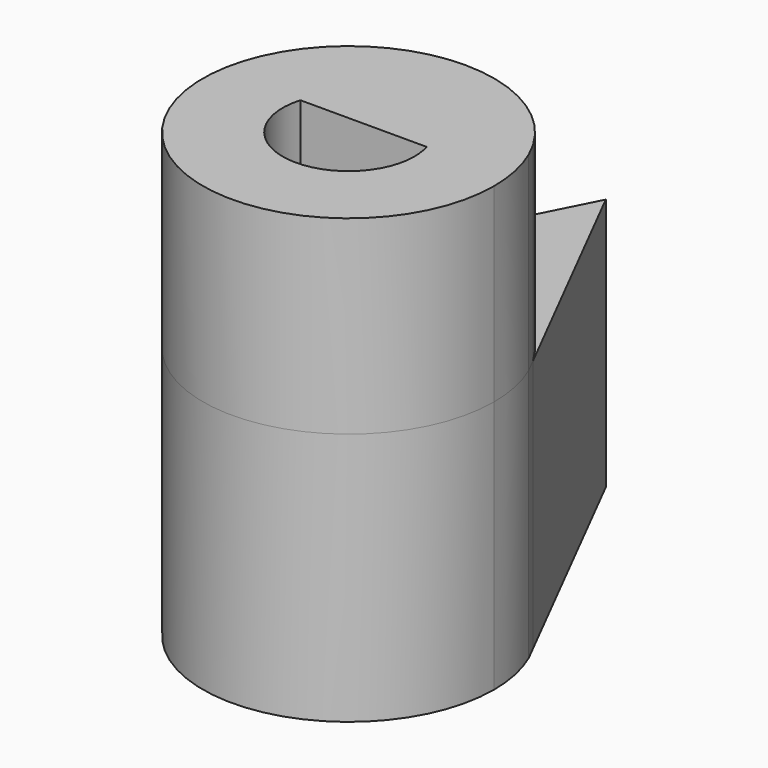
from build123d import *

# Parameters (mm, degrees)
F1_DEPTH = 9.525
F2_DEPTH = 12.7
F3_DEPTH = 9.525


# Not quite as in the source:
# - a feature names something its author has since deleted; it is built from what else it names
# - the program builds the solid bodies; features that only make, move or delete a surface that nothing else refers to are left out


with BuildPart() as f1:
    # F0 (on Top) → F1 (new body)
    with BuildSketch(Plane.XY):
        with BuildLine():
            ThreePointArc((-6.7061053414, 2.890442423), (-1.4756645952, -7.1518473315), (7.3025, 0))
            ThreePointArc((7.3025, 0), (7.1473488528, 1.4973011139), (6.6884881888, 2.9309779936))
            Line((6.6884881888, 2.9309779936), (6.3166219962, 3.6642588347))
            ThreePointArc((6.3166219962, 3.6642588347), (0.0208084361, 7.3024703532), (-6.2956369305, 3.7001975474))
            Line((-6.2956369305, 3.7001975474), (-6.7061053414, 2.890442423))
        make_face()
        with BuildLine():
            ThreePointArc((3.1654351928, 0.9398), (3.2676804469, 0.474835231), (3.302, 0))
            ThreePointArc((3.302, 0), (-0.474835231, -3.2676804469), (-3.1654351928, 0.9398))
            ThreePointArc((-3.1654351928, 0.9398), (0, 3.302), (3.1654351928, 0.9398))
        make_face(mode=Mode.SUBTRACT)
    extrude(amount=F1_DEPTH)

    # F0 (on Top) → F3 (join, through all)
    with BuildSketch(Plane.XY):
        with BuildLine():
            Line((-3.1654351928, 0.9398), (3.1654351928, 0.9398))
            ThreePointArc((3.1654351928, 0.9398), (0, 3.302), (-3.1654351928, 0.9398))
        make_face()
    extrude(amount=F3_DEPTH)


with BuildPart() as f2:
    # F0 (on Top) → F2 (new body)
    with BuildSketch(Plane.XY):
        with BuildLine():
            ThreePointArc((-6.7061053414, 2.890442423), (-1.4756645952, -7.1518473315), (7.3025, 0))
            ThreePointArc((7.3025, 0), (7.1473488528, 1.4973011139), (6.6884881888, 2.9309779936))
            Line((6.6884881888, 2.9309779936), (6.3166219962, 3.6642588347))
            ThreePointArc((6.3166219962, 3.6642588347), (0.0208084361, 7.3024703532), (-6.2956369305, 3.7001975474))
            Line((-6.2956369305, 3.7001975474), (-6.7061053414, 2.890442423))
        make_face()
        with BuildLine():
            ThreePointArc((3.1654351928, 0.9398), (3.2676804469, 0.474835231), (3.302, 0))
            ThreePointArc((3.302, 0), (-0.474835231, -3.2676804469), (-3.1654351928, 0.9398))
            ThreePointArc((-3.1654351928, 0.9398), (0, 3.302), (3.1654351928, 0.9398))
        make_face(mode=Mode.SUBTRACT)
        with BuildLine():
            ThreePointArc((-6.2956369305, 3.7001975474), (0.0208084361, 7.3024703532), (6.3166219962, 3.6642588347))
            Line((6.3166219962, 3.6642588347), (0, 16.1199700087))
            Line((0, 16.1199700087), (-6.2956369305, 3.7001975474))
        make_face()
    extrude(amount=-F2_DEPTH)


solid = Compound([f1.part, f2.part])
